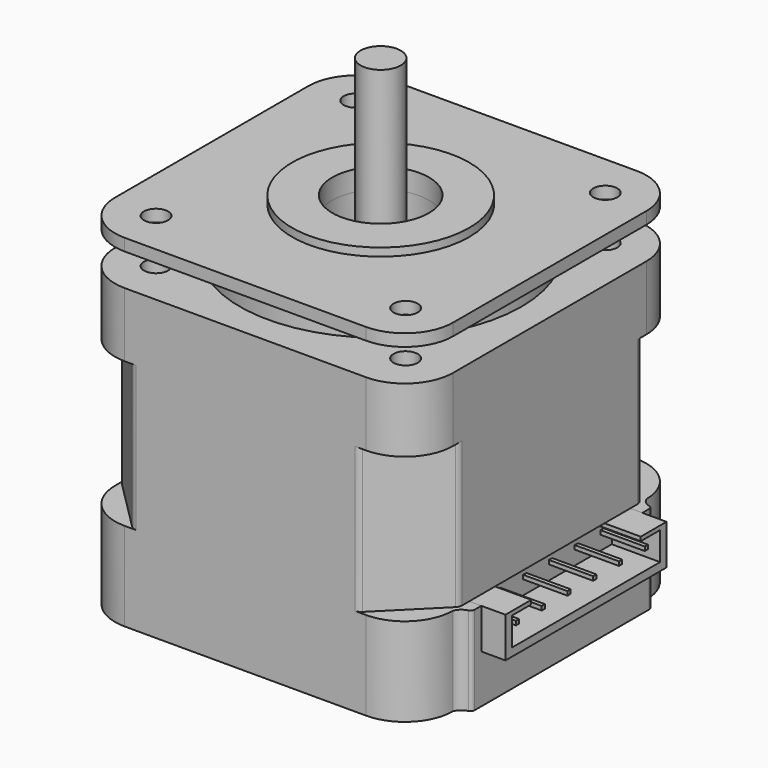
from build123d import *

# Parameters (mm, degrees)
F1_DEPTH  = 9
F2_R      = 1
F4_DEPTH  = 11
F5_R      = 5.99999
F6_R      = 0.5
F7_R      = 4.5
F8_DEPTH  = 5
F9_R      = 3
F10_DEPTH = 3
F12_DEPTH = 8
F13_R     = 6
F14_R     = 1.5
F15_DEPTH = 10
F16_R     = 17.5
F17_DEPTH = 4
F18_R     = 6
F19_DEPTH = 4
F20_R     = 2.5
F21_DEPTH = 21.5
F22_R     = 1.5
F22_R_2   = 17.5
F22_R_3   = 6
F23_DEPTH = 1.5
F24_R     = 11
F24_R_2   = 6
F25_DEPTH = 1
F26_W     = 25
F26_H     = 5
F27_DEPTH = 3
F29_DEPTH = 6
F30_W     = 0.5
F30_H     = 0.5
F31_DEPTH = 5.5


# Not quite as in the source:
# - a fillet or chamfer is up to 0.001 mm smaller than in the source, because OpenCascade refuses the exact size


with BuildPart() as f1:
    # F0 (on Top) → F1 (new body, symmetric)
    with BuildSketch(Plane.XY):
        Polygon((21, 14), (14, 21), (-14, 21), (-21, 14), (-21, -14), (-14, -21), (14, -21), (21, -14), align=None)
    extrude(amount=F1_DEPTH, both=True)

    # F2
    f2_edges = [f1.edges().sort_by_distance(p)[0] for p in [
        (-21, -14, 0),
        (-14, -21, 0),
        (14, -21, 0),
        (21, -14, 0),
        (21, 14, 0),
        (14, 21, 0),
        (-14, 21, 0),
        (-21, 14, 0),
    ]]
    fillet(f2_edges, radius=F2_R)

    # F3 (on face) → F4 (join)
    with BuildSketch(Plane(origin=(0, 0, -9), x_dir=(1, 0, 0), z_dir=(0, 0, -1))):
        with BuildLine():
            Line((13.5857864376, 21), (-13.5857864376, 21))
            ThreePointArc((-13.5857864376, 21), (-13.96846987, 20.9238795325), (-14.2928932188, 20.7071067812))
            Line((-14.2928932188, 20.7071067812), (-20.7071067812, 14.2928932188))
            ThreePointArc((-20.7071067812, 14.2928932188), (-20.9238795325, 13.96846987), (-21, 13.5857864376))
            Line((-21, 13.5857864376), (-21, -13.5857864376))
            ThreePointArc((-21, -13.5857864376), (-20.9238795325, -13.96846987), (-20.7071067812, -14.2928932188))
            Line((-20.7071067812, -14.2928932188), (-14.2928932188, -20.7071067812))
            ThreePointArc((-14.2928932188, -20.7071067812), (-13.96846987, -20.9238795325), (-13.5857864376, -21))
            Line((-13.5857864376, -21), (13.5857864376, -21))
            ThreePointArc((13.5857864376, -21), (13.96846987, -20.9238795325), (14.2928932188, -20.7071067812))
            Line((14.2928932188, -20.7071067812), (20.7071067812, -14.2928932188))
            ThreePointArc((20.7071067812, -14.2928932188), (20.9238795325, -13.96846987), (21, -13.5857864376))
            Line((21, -13.5857864376), (21, 13.5857864376))
            ThreePointArc((21, 13.5857864376), (20.9238795325, 13.96846987), (20.7071067812, 14.2928932188))
            Line((20.7071067812, 14.2928932188), (14.2928932188, 20.7071067812))
            ThreePointArc((14.2928932188, 20.7071067812), (13.96846987, 20.9238795325), (13.5857864376, 21))
        make_face()
        with BuildLine():
            ThreePointArc((14.2928932188, -20.7071067812), (13.96846987, -20.9238795325), (13.5857864376, -21))
            Line((13.5857864376, -21), (21, -21))
            Line((21, -21), (21, -15))
            Line((21, -15), (21, -14))
            Line((21, -14), (21, -13.5857864376))
            ThreePointArc((21, -13.5857864376), (20.9238795325, -13.96846987), (20.7071067812, -14.2928932188))
            Line((20.7071067812, -14.2928932188), (14.2928932188, -20.7071067812))
        make_face()
        with BuildLine():
            Line((-13.5857864376, 21), (-21, 21))
            Line((-21, 21), (-21, 13.5857864376))
            ThreePointArc((-21, 13.5857864376), (-20.9238795325, 13.96846987), (-20.7071067812, 14.2928932188))
            Line((-20.7071067812, 14.2928932188), (-14.2928932188, 20.7071067812))
            ThreePointArc((-14.2928932188, 20.7071067812), (-13.96846987, 20.9238795325), (-13.5857864376, 21))
        make_face()
        with BuildLine():
            Line((21, 21), (13.5857864376, 21))
            ThreePointArc((13.5857864376, 21), (13.96846987, 20.9238795325), (14.2928932188, 20.7071067812))
            Line((14.2928932188, 20.7071067812), (20.7071067812, 14.2928932188))
            ThreePointArc((20.7071067812, 14.2928932188), (20.9238795325, 13.96846987), (21, 13.5857864376))
            Line((21, 13.5857864376), (21, 14))
            Line((21, 14), (21, 15))
            Line((21, 15), (21, 21))
        make_face()
        with BuildLine():
            ThreePointArc((-20.7071067812, -14.2928932188), (-20.9238795325, -13.96846987), (-21, -13.5857864376))
            Line((-21, -13.5857864376), (-21, -21))
            Line((-21, -21), (-13.5857864376, -21))
            ThreePointArc((-13.5857864376, -21), (-13.96846987, -20.9238795325), (-14.2928932188, -20.7071067812))
            Line((-14.2928932188, -20.7071067812), (-20.7071067812, -14.2928932188))
        make_face()
        Polygon((22.5, 14), (21, 14), (21, 13.5857864376), (21, -13.5857864376), (21, -14), (22.5, -14), align=None)
        with BuildLine():
            ThreePointArc((22.5, 14), (21.5986121811, 14.2729182717), (21, 15))
            Line((21, 15), (21, 14))
            Line((21, 14), (22.5, 14))
        make_face()
        with BuildLine():
            ThreePointArc((21, -15), (21.5986121811, -14.2729182717), (22.5, -14))
            Line((22.5, -14), (21, -14))
            Line((21, -14), (21, -15))
        make_face()
    extrude(amount=F4_DEPTH)

    # F5 (radius 6 in the source; OpenCascade refuses exactly that, so slightly less here)
    f5_edges = [f1.edges().sort_by_distance(p)[0] for p in [
        (21, -21, -14.5),
        (21, 21, -14.5),
        (-21, 21, -14.5),
        (-21, -21, -14.5),
    ]]
    fillet(f5_edges, radius=F5_R)

    # F6
    f6_edges = [f1.edges().sort_by_distance(p)[0] for p in [
        (22.5, -14, -14.5),
        (22.5, 14, -14.5),
    ]]
    fillet(f6_edges, radius=F6_R)

    # F7 (on face) → F8 (cut)
    with BuildSketch(Plane(origin=(0, 0, -20), x_dir=(1, 0, 0), z_dir=(0, 0, -1))):
        Circle(F7_R)
    extrude(amount=-F8_DEPTH, mode=Mode.SUBTRACT)

    # F9 (on face) → F10 (cut)
    with BuildSketch(Plane(origin=(0, 0, -20), x_dir=(1, 0, 0), z_dir=(0, 0, -1))):
        with Locations((15.5, 15.5)):
            Circle(F9_R)
        with Locations((15.5, -15.5)):
            Circle(F9_R)
        with Locations((-15.5, -15.5)):
            Circle(F9_R)
        with Locations((-15.5, 15.5)):
            Circle(F9_R)
    extrude(amount=-F10_DEPTH, mode=Mode.SUBTRACT)

    # F11 (on face) → F12 (join)
    with BuildSketch(Plane.XY.offset(9)):
        with BuildLine():
            Line((-13.5857864376, -21), (13.5857864376, -21))
            ThreePointArc((13.5857864376, -21), (13.96846987, -20.9238795325), (14.2928932188, -20.7071067812))
            Line((14.2928932188, -20.7071067812), (20.7071067812, -14.2928932188))
            ThreePointArc((20.7071067812, -14.2928932188), (20.9238795325, -13.96846987), (21, -13.5857864376))
            Line((21, -13.5857864376), (21, 13.5857864376))
            ThreePointArc((21, 13.5857864376), (20.9238795325, 13.96846987), (20.7071067812, 14.2928932188))
            Line((20.7071067812, 14.2928932188), (14.2928932188, 20.7071067812))
            ThreePointArc((14.2928932188, 20.7071067812), (13.96846987, 20.9238795325), (13.5857864376, 21))
            Line((13.5857864376, 21), (-13.5857864376, 21))
            ThreePointArc((-13.5857864376, 21), (-13.96846987, 20.9238795325), (-14.2928932188, 20.7071067812))
            Line((-14.2928932188, 20.7071067812), (-20.7071067812, 14.2928932188))
            ThreePointArc((-20.7071067812, 14.2928932188), (-20.9238795325, 13.96846987), (-21, 13.5857864376))
            Line((-21, 13.5857864376), (-21, -13.5857864376))
            ThreePointArc((-21, -13.5857864376), (-20.9238795325, -13.96846987), (-20.7071067812, -14.2928932188))
            Line((-20.7071067812, -14.2928932188), (-14.2928932188, -20.7071067812))
            ThreePointArc((-14.2928932188, -20.7071067812), (-13.96846987, -20.9238795325), (-13.5857864376, -21))
        make_face()
        with BuildLine():
            Line((-21, 21), (-21, 13.5857864376))
            ThreePointArc((-21, 13.5857864376), (-20.9238795325, 13.96846987), (-20.7071067812, 14.2928932188))
            Line((-20.7071067812, 14.2928932188), (-14.2928932188, 20.7071067812))
            ThreePointArc((-14.2928932188, 20.7071067812), (-13.96846987, 20.9238795325), (-13.5857864376, 21))
            Line((-13.5857864376, 21), (-21, 21))
        make_face()
        with BuildLine():
            ThreePointArc((20.7071067812, 14.2928932188), (20.9238795325, 13.96846987), (21, 13.5857864376))
            Line((21, 13.5857864376), (21, 21))
            Line((21, 21), (13.5857864376, 21))
            ThreePointArc((13.5857864376, 21), (13.96846987, 20.9238795325), (14.2928932188, 20.7071067812))
            Line((14.2928932188, 20.7071067812), (20.7071067812, 14.2928932188))
        make_face()
        with BuildLine():
            Line((13.5857864376, -21), (21, -21))
            Line((21, -21), (21, -13.5857864376))
            ThreePointArc((21, -13.5857864376), (20.9238795325, -13.96846987), (20.7071067812, -14.2928932188))
            Line((20.7071067812, -14.2928932188), (14.2928932188, -20.7071067812))
            ThreePointArc((14.2928932188, -20.7071067812), (13.96846987, -20.9238795325), (13.5857864376, -21))
        make_face()
        with BuildLine():
            Line((-21, -21), (-13.5857864376, -21))
            ThreePointArc((-13.5857864376, -21), (-13.96846987, -20.9238795325), (-14.2928932188, -20.7071067812))
            Line((-14.2928932188, -20.7071067812), (-20.7071067812, -14.2928932188))
            ThreePointArc((-20.7071067812, -14.2928932188), (-20.9238795325, -13.96846987), (-21, -13.5857864376))
            Line((-21, -13.5857864376), (-21, -21))
        make_face()
    extrude(amount=F12_DEPTH)

    # F13
    f13_edges = [f1.edges().sort_by_distance(p)[0] for p in [
        (-21, -21, 13),
        (21, -21, 13),
        (21, 21, 13),
        (-21, 21, 13),
    ]]
    fillet(f13_edges, radius=F13_R)

    # F14 (on face) → F15 (cut)
    with BuildSketch(Plane.XY.offset(17)):
        with Locations((15.5, 15.5)):
            Circle(F14_R)
        with Locations((15.5, -15.5)):
            Circle(F14_R)
        with Locations((-15.5, -15.5)):
            Circle(F14_R)
        with Locations((-15.5, 15.5)):
            Circle(F14_R)
    extrude(amount=-F15_DEPTH, mode=Mode.SUBTRACT)

    # F20 (on face) → F21 (join)
    with BuildSketch(Plane.XY.offset(17)):
        Circle(F20_R)
    extrude(amount=F21_DEPTH)

    # F26 (on face) → F27 (cut)
    with BuildSketch(Plane.YZ.offset(22.5)):
        with Locations((1.0448e-06, -11.5)):
            Rectangle(F26_W, F26_H)
    extrude(amount=-F27_DEPTH, mode=Mode.SUBTRACT)

    # F30 (on face) → F31 (join)
    with BuildSketch(Plane.YZ.offset(19.5)):
        with Locations((-9.9999989552, -11)):
            Rectangle(F30_W, F30_H)
        with Locations((-5.9999989552, -11)):
            Rectangle(F30_W, F30_H)
        with Locations((-1.9999989552, -11)):
            Rectangle(F30_W, F30_H)
        with Locations((2.0000010448, -11)):
            Rectangle(F30_W, F30_H)
        with Locations((6.0000010448, -11)):
            Rectangle(F30_W, F30_H)
        with Locations((10.0000010448, -11)):
            Rectangle(F30_W, F30_H)
    extrude(amount=F31_DEPTH)


with BuildPart() as f17:
    # F16 (on face) → F17 (new body)
    with BuildSketch(Plane.XY.offset(17)):
        Circle(F16_R)
    extrude(amount=F17_DEPTH)

    # F18 (on face) → F19 (cut)
    with BuildSketch(Plane.XY.offset(21)):
        Circle(F18_R)
    extrude(amount=-F19_DEPTH, mode=Mode.SUBTRACT)


with BuildPart() as f23:
    # F22 (on face) → F23 (new body)
    with BuildSketch(Plane.XY.offset(21)):
        with BuildLine():
            ThreePointArc((-21, -15), (-19.2426406871, -19.2426406871), (-15, -21))
            Line((-15, -21), (15, -21))
            ThreePointArc((15, -21), (19.2426406871, -19.2426406871), (21, -15))
            Line((21, -15), (21, 15))
            ThreePointArc((21, 15), (19.2426406871, 19.2426406871), (15, 21))
            Line((15, 21), (-15, 21))
            ThreePointArc((-15, 21), (-19.2426406871, 19.2426406871), (-21, 15))
            Line((-21, 15), (-21, -15))
        make_face()
        with Locations((-15.5, -15.5)):
            Circle(F22_R, mode=Mode.SUBTRACT)
        with Locations((15.5, -15.5)):
            Circle(F22_R, mode=Mode.SUBTRACT)
        with Locations((-15.5, 15.5)):
            Circle(F22_R, mode=Mode.SUBTRACT)
        Circle(F22_R_2, mode=Mode.SUBTRACT)
        with Locations((15.5, 15.5)):
            Circle(F22_R, mode=Mode.SUBTRACT)
        Circle(F22_R_2)
        Circle(F22_R_3, mode=Mode.SUBTRACT)
    extrude(amount=F23_DEPTH)

    # F24 (on face) → F25 (join)
    with BuildSketch(Plane.XY.offset(22.5)):
        Circle(F24_R)
        Circle(F24_R_2, mode=Mode.SUBTRACT)
    extrude(amount=F25_DEPTH)


with BuildPart() as f29:
    # F28 (on face) → F29 (new body)
    with BuildSketch(Plane.YZ.offset(19.5)):
        Polygon((-8.4999989552, -9), (-12.4999989552, -9), (-12.4999989552, -14), (12.5000010448, -14), (12.5000010448, -9), (8.4999989552, -9), (8.4999989552, -9.5), (11.5000010448, -9.5), (11.5000010448, -13), (-11.4999989552, -13), (-11.4999989552, -9.5), (-8.4999989552, -9.5), align=None)
    extrude(amount=F29_DEPTH)


solid = Compound([f1.part, f17.part, f23.part, f29.part])
